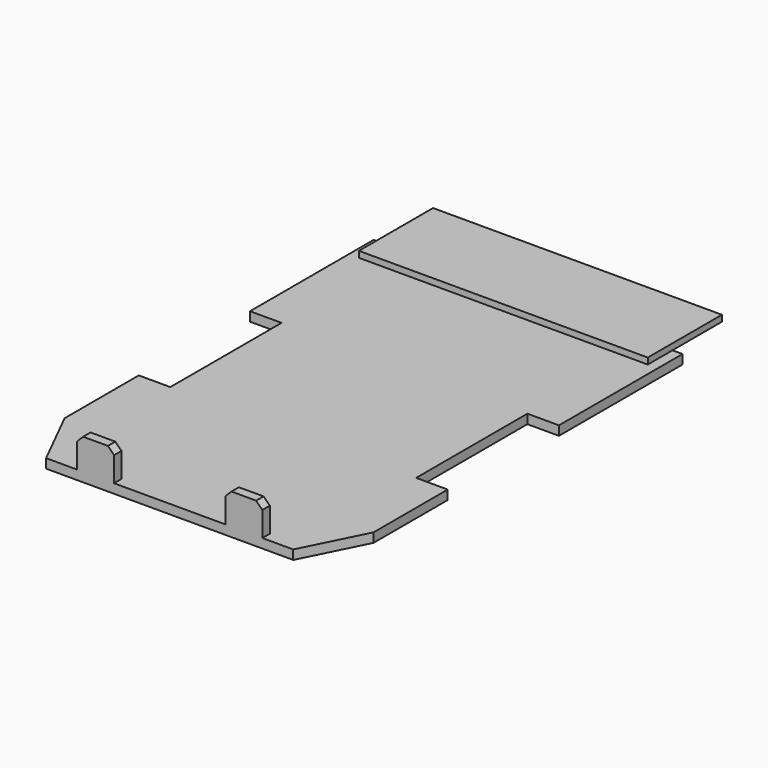
from build123d import *

# Parameters (mm, degrees)
F1_DEPTH = 3
F2_W     = 12
F2_H     = 3
F3_DEPTH = 10
F4_SIZE  = 2
F5_W     = 93.5
F5_H     = 30
F6_DEPTH = 2


# Not quite as in the source:
# - a feature names something its author has since deleted; it is built from what else it names


with BuildPart() as f1:
    # F0 (on Top) → F1 (new body)
    with BuildSketch(Plane.XY):
        Polygon((50, -18.8796229661), (-50, -18.8796229661), (-50, -68.8796229661), (-39.780523628, -68.8796229661), (-39.780523628, -113.8796229661), (-50, -113.8796229661), (-50, -143.8796229661), (-40, -163.8796229661), (40, -163.8796229661), (50, -143.8796229661), (50, -113.8796229661), (39.780523628, -113.8796229661), (39.780523628, -68.8796229661), (50, -68.8796229661), align=None)
    extrude(amount=F1_DEPTH)

    # F2 (on face) → F3 (join)
    with BuildSketch(Plane.XY.offset(3)):
        with Locations((-24, -162.3796229661)):
            Rectangle(F2_W, F2_H)
        with Locations((24, -162.3796229661)):
            Rectangle(F2_W, F2_H)
    extrude(amount=F3_DEPTH)

    # F4
    f4_edges = [f1.edges().sort_by_distance(p)[0] for p in [
        (-18, -162.379623, 13),
        (-30, -162.379623, 13),
        (30, -162.379623, 13),
        (18, -162.379623, 13),
    ]]
    chamfer(f4_edges, length=F4_SIZE)

    # F5 (on face) → F6 (join)
    with BuildSketch(Plane.XY.offset(3)):
        with Locations((0, -13.8796229661)):
            Rectangle(F5_W, F5_H)
    extrude(amount=F6_DEPTH)


solid = f1.part
